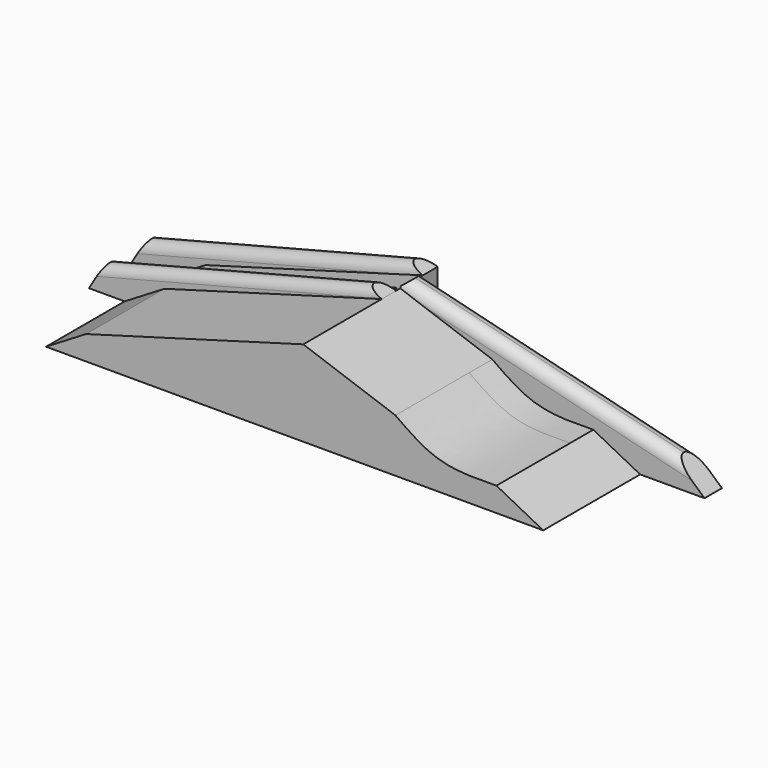
from build123d import *

# Parameters (mm, degrees)
F1_DEPTH      = 68.834
F3_DEPTH      = 56.642
F4_DEPTH      = 21.59
F6_DEPTH      = 16.256
F7_T1_DEPTH   = 134.6089194051
F8_SIZE       = 5.08
F9_T4_DEPTH   = 246.1695934192
F9_T9_DEPTH   = 246.1695934192
F11_DEPTH     = 13.97
F12_T1_DEPTH  = 239.1129526059
F12_T6_DEPTH  = 239.1129526059
F13_W         = 8.2417714845
F13_H         = 1.1003240943
F14_DEPTH     = 1.524
F16_DEPTH     = 13.208
F17_T1_DEPTH  = 236.9807138407
F17_T6_DEPTH  = 236.9807138407
F17_T12_DEPTH = 236.9807138407
F17_T18_DEPTH = 236.9807138407


# Not quite as in the source:
# - a fillet or chamfer that OpenCascade refuses, or shapes differently, is made with other operations: its cross-section is extruded or revolved along the edge and cut away or added


with BuildPart() as f1:
    # F0 (on Front) → F1 (new body)
    with BuildSketch(Plane.XZ):
        with BuildLine():
            Line((-134.6334815025, -70.4434812069), (236.5282326937, -70.4434812069))
            Line((236.5282326937, -70.4434812069), (201.5823870897, -52.4187758565))
            add(Edge.make_bspline(
                [(201.5823870897, -52.4187758565), (186.6945113423, -52.7201094998), (157.86128429, -53.3036998994), (136.5029788289, -38.0790520799), (126.1729151011, -30.7155661285)],
                knots=[0, 0, 0, 0, 0.5163444147, 1, 1, 1, 1], degree=3))
            Line((126.1729151011, -30.7155661285), (57.3847740889, -6.4373956993))
            Line((57.3847740889, -6.4373956993), (-104.8375442624, -52.4187758565))
            Line((-104.8375442624, -52.4187758565), (-134.6334815025, -70.4434812069))
        make_face()
    extrude(amount=-F1_DEPTH)

    # F2 (on face) → F3 (join)
    with BuildSketch(Plane(origin=(0, 68.834, 0), x_dir=(-1, 0, 0), z_dir=(0, 1, 0))):
        Polygon((104.8375442624, -52.4187758565), (-57.3847740889, -6.4373956993), (-57.3847740889, -70.4434812069), (134.6334815025, -70.4434812069), align=None)
    extrude(amount=F3_DEPTH)

    # F4 (add): a face of the model
    f4_faces = [f1.faces().sort_by_distance(p)[0] for p in [
        (117.597457412, 68.834, -49.4942566091),
    ]]
    extrude(f4_faces, amount=F4_DEPTH)

    # F5 (on face) → F6 (join)
    with BuildSketch(Plane(origin=(0, 90.424, 0), x_dir=(-1, 0, 0), z_dir=(0, 1, 0))):
        Polygon((-284.8027348518, -56.1655424535), (-284.8027348518, -70.4434812069), (-57.3847740889, -70.4434812069), (-57.3847740889, 0), align=None)
    extrude(amount=F6_DEPTH)

    # F7: chamfer of 22.86 x 14.478 on 1 edges, made by hand

    # F7_s2 → F7_t1 (cut)
    with BuildSketch(Plane.XZ.offset(-165.8564597025)):
        Polygon((262.6095480908, -50.6844785612), (284.8027348518, -70.6435424535), (284.8027348518, -56.1655424535), align=None)
    extrude(amount=F7_T1_DEPTH, mode=Mode.SUBTRACT)

    # F8
    f8_edges = [f1.edges().sort_by_distance(p)[0] for p in [
        (57.384774, 98.552, 0),
    ]]
    chamfer(f8_edges, length=F8_SIZE)

    # F9: fillet of radius 7.971733183 on 2 edges, made by hand


with BuildPart() as f9_tool2:
    # F9_s3 → F9_t4 (new body)
    with BuildSketch(Plane(origin=(39.6696512747, 0, -9.7972362223), x_dir=(0, 1, 0), z_dir=(0.970830567, 0, -0.2397665745))):
        with BuildLine():
            ThreePointArc((106.68, 5.7872175269), (104.3451334085, 11.4240841184), (98.708266817, 13.7589507099))
            Line((98.708266817, 13.7589507099), (106.68, 13.7589507099))
            Line((106.68, 13.7589507099), (106.68, 5.7872175269))
        make_face()
    extrude(amount=F9_T4_DEPTH)

    split(bisect_by=Plane.YZ.offset(57.3847740889), keep=Keep.TOP)


with BuildPart() as f1_1:
    add(f1.part)

    # F9_t1: cut F9_tool2
    add(f9_tool2.part, mode=Mode.SUBTRACT)


with BuildPart() as f9_tool7:
    # F9_s8 → F9_t9 (new body)
    with BuildSketch(Plane(origin=(39.6696512747, 0, -9.7972362223), x_dir=(0, 1, 0), z_dir=(0.970830567, 0, -0.2397665745))):
        with BuildLine():
            ThreePointArc((90.424, 5.7872175269), (92.7588665915, 11.4240841184), (98.395733183, 13.7589507099))
            Line((98.395733183, 13.7589507099), (90.424, 13.7589507099))
            Line((90.424, 13.7589507099), (90.424, 5.7872175269))
        make_face()
    extrude(amount=F9_T9_DEPTH)

    split(bisect_by=Plane(origin=(4.3361166105, 0, 12.285662205), x_dir=(0, 1, 0), z_dir=(0.3328201545, 0, 0.9429903206)), keep=Keep.TOP)


with BuildPart() as f1_2:
    add(f1_1.part)

    # F9_t6: cut F9_tool7
    add(f9_tool7.part, mode=Mode.SUBTRACT)

    # F10 (on face) → F11 (join)
    with BuildSketch(Plane(origin=(0, 125.476, 0), x_dir=(-1, 0, 0), z_dir=(0, 1, 0))):
        Polygon((-45.8267219365, -2.2306151222), (-57.3847740889, -6.4373956993), (104.8375442624, -52.4187758565), (134.6334815025, -70.4434812069), (161.1742377281, -70.4434812069), (150.1698791981, -52.4187758565), align=None)
    extrude(amount=-F11_DEPTH)

    # F12: fillet of radius 7.3585229381 on 2 edges, made by hand

    # F12_s2 → F12_t1 (cut)
    with BuildSketch(Plane(origin=(-171.3471837913, 0, -43.8762710766), x_dir=(0, 1, 0), z_dir=(0.9687439392, 0, 0.2480628554))):
        with BuildLine():
            ThreePointArc((118.1174770619, -13.5288023788), (123.3207385309, -15.6840638479), (125.476, -20.8873253169))
            Line((125.476, -20.8873253169), (125.476, -13.5288023788))
            Line((125.476, -13.5288023788), (118.1174770619, -13.5288023788))
        make_face()
    extrude(amount=F12_T1_DEPTH, mode=Mode.SUBTRACT)


with BuildPart() as f12_tool4:
    # F12_s5 → F12_t6 (new body)
    with BuildSketch(Plane(origin=(-171.3471837913, 0, -43.8762710766), x_dir=(0, 1, 0), z_dir=(0.9687439392, 0, 0.2480628554))):
        with BuildLine():
            ThreePointArc((118.8645229381, -13.5288023788), (113.6612614691, -15.6840638479), (111.506, -20.8873253169))
            Line((111.506, -20.8873253169), (111.506, -13.5288023788))
            Line((111.506, -13.5288023788), (118.8645229381, -13.5288023788))
        make_face()
    extrude(amount=F12_T6_DEPTH)

    split(bisect_by=Plane(origin=(5.9565096776, 0, -21.0145673287), x_dir=(0, 1, 0), z_dir=(-0.272703532, 0, 0.9620981154)), keep=Keep.TOP)


with BuildPart() as f1_3:
    add(f1_2.part)

    # F12_t3: cut F12_tool4
    add(f12_tool4.part, mode=Mode.SUBTRACT)

    # F13 (on face) → F14 (join)
    with BuildSketch(Plane(origin=(5.9565096776, 0, -21.0145673287), x_dir=(0.9620981154, 0, 0.272703532), z_dir=(-0.272703532, 0, 0.9620981154))):
        with Locations((49.3333967155, 86.9543515146)):
            Rectangle(F13_W, F13_H)
    extrude(amount=F14_DEPTH)

    # F15 (on face) → F16 (join)
    with BuildSketch(Plane.XZ.offset(-86.4041894674)):
        Polygon((-104.8238277435, -52.4797327816), (57.3847740889, -6.4373956993), (46.4603118598, -2.0644166507), (-150.4420638084, -52.4797327816), (-161.1757725477, -70.3692361712), (-134.1178864241, -70.3692361712), align=None)
    extrude(amount=F16_DEPTH)

    # F17: fillet of radius 6.7453126933 on 2 edges, made by hand

    # F17_s2 → F17_t1 (cut)
    with BuildSketch(Plane(origin=(59.4421171299, 0, 15.219690044), x_dir=(0, 1, 0), z_dir=(-0.9687495941, 0, -0.2480407708))):
        with BuildLine():
            ThreePointArc((73.1961894674, 20.2692670518), (75.1718458141, 15.4996107052), (79.9415021607, 13.5239543585))
            Line((79.9415021607, 13.5239543585), (73.1961894674, 13.5239543585))
            Line((73.1961894674, 13.5239543585), (73.1961894674, 20.2692670518))
        make_face()
    extrude(amount=F17_T1_DEPTH, mode=Mode.SUBTRACT)


with BuildPart() as f17_tool4:
    # F17_s5 → F17_t6 (new body)
    with BuildSketch(Plane(origin=(59.4421171299, 0, 15.219690044), x_dir=(0, 1, 0), z_dir=(-0.9687495941, 0, -0.2480407708))):
        with BuildLine():
            ThreePointArc((86.4041894674, 20.2692670518), (84.4285331208, 15.4996107052), (79.6588767742, 13.5239543585))
            Line((79.6588767742, 13.5239543585), (86.4041894674, 13.5239543585))
            Line((86.4041894674, 13.5239543585), (86.4041894674, 20.2692670518))
        make_face()
    extrude(amount=F17_T6_DEPTH)

    split(bisect_by=Plane(origin=(43.4988715987, 0, 12.3296114352), x_dir=(0, 1, 0), z_dir=(0.9620981154, 0, 0.272703532)), keep=Keep.TOP)

    split(bisect_by=Plane(origin=(5.5409094947, 0, -19.5483298008), x_dir=(0, 1, 0), z_dir=(-0.272703532, 0, 0.9620981154)), keep=Keep.TOP)


with BuildPart() as f1_4:
    add(f1_3.part)

    # F17_t3: cut F17_tool4
    add(f17_tool4.part, mode=Mode.SUBTRACT)


with BuildPart() as f17_tool10:
    # F17_s11 → F17_t12 (new body)
    with BuildSketch(Plane(origin=(59.4421171299, 0, 15.219690044), x_dir=(0, 1, 0), z_dir=(-0.9687495941, 0, -0.2480407708))):
        with BuildLine():
            ThreePointArc((86.4041894674, 20.2692670518), (84.4285331208, 15.4996107052), (79.6588767742, 13.5239543585))
            Line((79.6588767742, 13.5239543585), (86.4041894674, 13.5239543585))
            Line((86.4041894674, 13.5239543585), (86.4041894674, 20.2692670518))
        make_face()
    extrude(amount=F17_T12_DEPTH)

    split(bisect_by=Plane(origin=(43.4988715987, 0, 12.3296114352), x_dir=(0, 1, 0), z_dir=(-0.9620981154, 0, -0.272703532)), keep=Keep.TOP)

    split(bisect_by=Plane(origin=(5.5409094947, 0, -19.5483298008), x_dir=(0, 1, 0), z_dir=(0.272703532, 0, -0.9620981154)), keep=Keep.TOP)


with BuildPart() as f1_5:
    add(f1_4.part)

    # F17_t9: cut F17_tool10
    add(f17_tool10.part, mode=Mode.SUBTRACT)


with BuildPart() as f17_tool16:
    # F17_s17 → F17_t18 (new body)
    with BuildSketch(Plane(origin=(59.4421171299, 0, 15.219690044), x_dir=(0, 1, 0), z_dir=(-0.9687495941, 0, -0.2480407708))):
        with BuildLine():
            ThreePointArc((86.4041894674, 20.2692670518), (84.4285331208, 15.4996107052), (79.6588767742, 13.5239543585))
            Line((79.6588767742, 13.5239543585), (86.4041894674, 13.5239543585))
            Line((86.4041894674, 13.5239543585), (86.4041894674, 20.2692670518))
        make_face()
    extrude(amount=F17_T18_DEPTH)

    split(bisect_by=Plane(origin=(43.4988715987, 0, 12.3296114352), x_dir=(0, 1, 0), z_dir=(-0.9620981154, 0, -0.272703532)), keep=Keep.TOP)

    split(bisect_by=Plane(origin=(5.5409094947, 0, -19.5483298008), x_dir=(0, 1, 0), z_dir=(-0.272703532, 0, 0.9620981154)), keep=Keep.TOP)


with BuildPart() as f1_6:
    add(f1_5.part)

    # F17_t15: cut F17_tool16
    add(f17_tool16.part, mode=Mode.SUBTRACT)


solid = f1_6.part
